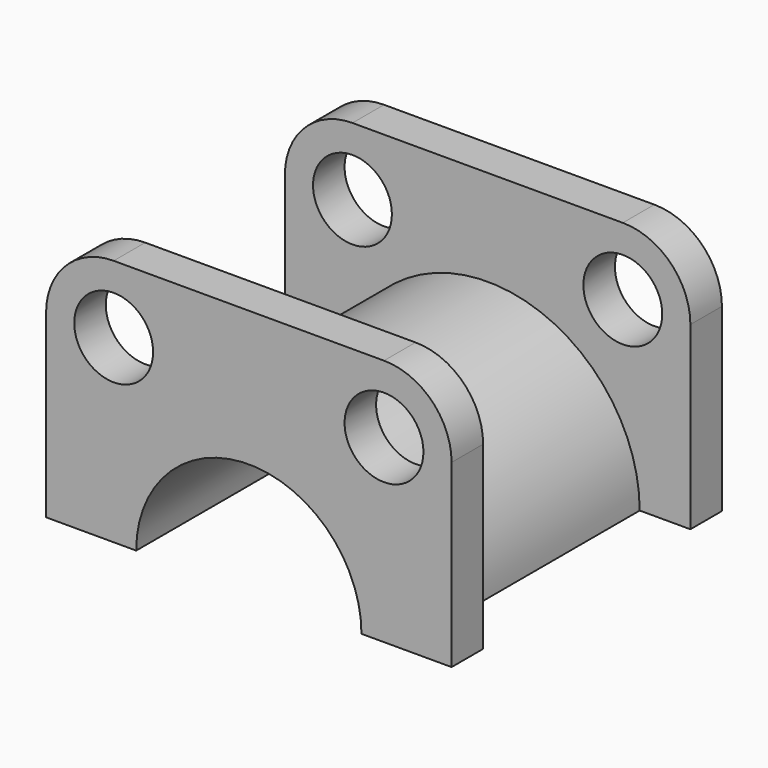
from build123d import *

# Parameters (mm, degrees)
F1_DEPTH = 95.25
F0_R     = 11.1125
F2_DEPTH = 11.1125
F3_R     = 11.1125
F4_DEPTH = 11.1125
F5_R     = 19.05


with BuildPart() as f1:
    # F0 (on Front) → F1 (new body)
    with BuildSketch(Plane.XZ):
        with BuildLine():
            Line((31.75, 0), (42.8625, 0))
            ThreePointArc((42.8625, 0), (0, 42.8625), (-42.8625, 0))
            Line((-42.8625, 0), (-31.75, 0))
            ThreePointArc((-31.75, 0), (0, 31.75), (31.75, 0))
        make_face()
    extrude(amount=F1_DEPTH)

    # F0 (on Front) → F2 (join)
    with BuildSketch(Plane.XZ):
        with BuildLine():
            ThreePointArc((-42.8625, 0), (0, 42.8625), (42.8625, 0))
            Line((42.8625, 0), (57.15, 0))
            Line((57.15, 0), (57.15, 69.85))
            Line((57.15, 69.85), (-57.15, 69.85))
            Line((-57.15, 69.85), (-57.15, 0))
            Line((-57.15, 0), (-42.8625, 0))
        make_face()
        with Locations((-38.1, 50.8)):
            Circle(F0_R, mode=Mode.SUBTRACT)
        with Locations((38.1, 50.8)):
            Circle(F0_R, mode=Mode.SUBTRACT)
    extrude(amount=F2_DEPTH)

    # F3 (on face) → F4 (join)
    with BuildSketch(Plane.XZ.offset(95.25)):
        with BuildLine():
            ThreePointArc((-42.8625, 0), (0, 42.8625), (42.8625, 0))
            Line((42.8625, 0), (57.15, 0))
            Line((57.15, 0), (57.15, 69.85))
            Line((57.15, 69.85), (-57.15, 69.85))
            Line((-57.15, 69.85), (-57.15, 0))
            Line((-57.15, 0), (-42.8625, 0))
        make_face()
        with Locations((-38.1, 50.8)):
            Circle(F3_R, mode=Mode.SUBTRACT)
        with Locations((38.1, 50.8)):
            Circle(F3_R, mode=Mode.SUBTRACT)
    extrude(amount=-F4_DEPTH)

    # F5
    f5_edges = [f1.edges().sort_by_distance(p)[0] for p in [
        (57.15, -89.69375, 69.85),
        (-57.15, -5.55625, 69.85),
        (-57.15, -89.69375, 69.85),
        (57.15, -5.55625, 69.85),
    ]]
    fillet(f5_edges, radius=F5_R)


solid = f1.part
